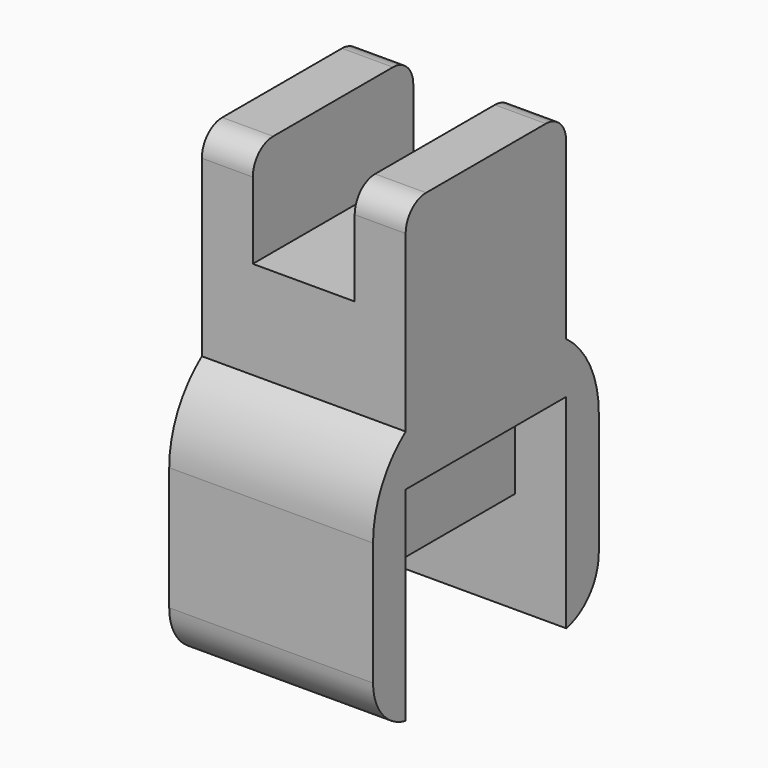
from build123d import *

# Parameters (mm, degrees)
F0_W          = 5.08
F0_H          = 9.99998
F1_DEPTH      = 12.5
F2_W          = 9.99998
F2_H          = 7.42
F3_DEPTH      = 2.54
F4_W          = 9.99998
F4_H          = 7.42
F5_DEPTH      = 2.54
F6_W          = 2.54
F6_H          = 9.99998
F7_DEPTH      = 5.08
F8_W          = 10.16
F8_H          = 2.032
F9_DEPTH      = 5.08
F9_DEPTH_BACK = 7.62
F10_T1_DEPTH  = 30.48
F11_R         = 1.27
F12_T1_DEPTH  = 22.6034078934


# Not quite as in the source:
# - a fillet or chamfer that OpenCascade refuses, or shapes differently, is made with other operations: its cross-section is extruded or revolved along the edge and cut away or added


with BuildPart() as f1:
    # F0 (on Top) → F1 (new body)
    with BuildSketch(Plane.XY):
        with Locations((2.54, 4.99999)):
            Rectangle(F0_W, F0_H)
    extrude(amount=F1_DEPTH)

    # F2 (on face) → F3 (join)
    with BuildSketch(Plane(origin=(0, 0, 0), x_dir=(0, -1, 0), z_dir=(-1, 0, 0))):
        with Locations((-4.99999, 8.79)):
            Rectangle(F2_W, F2_H)
    extrude(amount=F3_DEPTH)

    # F4 (on face) → F5 (join)
    with BuildSketch(Plane.YZ.offset(5.08)):
        with Locations((4.99999, 8.79)):
            Rectangle(F4_W, F4_H)
    extrude(amount=F5_DEPTH)

    # F6 (on face) → F7 (join)
    with BuildSketch(Plane.XY.offset(12.5)):
        with Locations((-1.27, 4.99999)):
            Rectangle(F6_W, F6_H)
        with Locations((6.35, 4.99999)):
            Rectangle(F6_W, F6_H)
    extrude(amount=F7_DEPTH)

    # F8 (on face) → F9 (join, two sides)
    with BuildSketch(Plane(origin=(0, 0, 0), x_dir=(1, 0, 0), z_dir=(0, 0, -1))) as f9_sk:
        with Locations((2.54, 1.016)):
            Rectangle(F8_W, F8_H)
        with Locations((2.54, -11.01598)):
            Rectangle(F8_W, F8_H)
    extrude(amount=F9_DEPTH)
    extrude(f9_sk.sketch, amount=-F9_DEPTH_BACK)

    # F10: fillet of radius 5.08 on 2 edges, made by hand

    # F10_s2 → F10_t1 (cut)
    with BuildSketch(Plane.YZ.offset(-12.7)):
        with BuildLine():
            ThreePointArc((0, 7.62), (-1.4956901303, 5.8278450651), (-2.032, 3.556))
            Line((-2.032, 3.556), (-2.032, 7.62))
            Line((-2.032, 7.62), (0, 7.62))
        make_face()
        with BuildLine():
            ThreePointArc((12.03198, 3.556), (11.4956701303, 5.8278450651), (9.99998, 7.62))
            Line((9.99998, 7.62), (12.03198, 7.62))
            Line((12.03198, 7.62), (12.03198, 3.556))
        make_face()
    extrude(amount=F10_T1_DEPTH, mode=Mode.SUBTRACT)

    # F11
    f11_edges = [f1.edges().sort_by_distance(p)[0] for p in [
        (-1.27, 0, 17.58),
        (6.35, 0, 17.58),
        (6.35, 9.99998, 17.58),
        (-1.27, 9.99998, 17.58),
    ]]
    fillet(f11_edges, radius=F11_R)

    # F12: fillet of radius 2.54 on 2 edges, made by hand

    # F12_s2 → F12_t1 (cut)
    with BuildSketch(Plane.YZ.offset(-8.7617039467)):
        with BuildLine():
            ThreePointArc((-2.032, -2.5913184213), (-1.4594755399, -4.1977554727), (0, -5.08))
            Line((0, -5.08), (-2.032, -5.08))
            Line((-2.032, -5.08), (-2.032, -2.5913184213))
        make_face()
        with BuildLine():
            ThreePointArc((12.03198, -2.5913184213), (11.4594555399, -4.1977554727), (9.99998, -5.08))
            Line((9.99998, -5.08), (12.03198, -5.08))
            Line((12.03198, -5.08), (12.03198, -2.5913184213))
        make_face()
    extrude(amount=F12_T1_DEPTH, mode=Mode.SUBTRACT)


solid = f1.part
